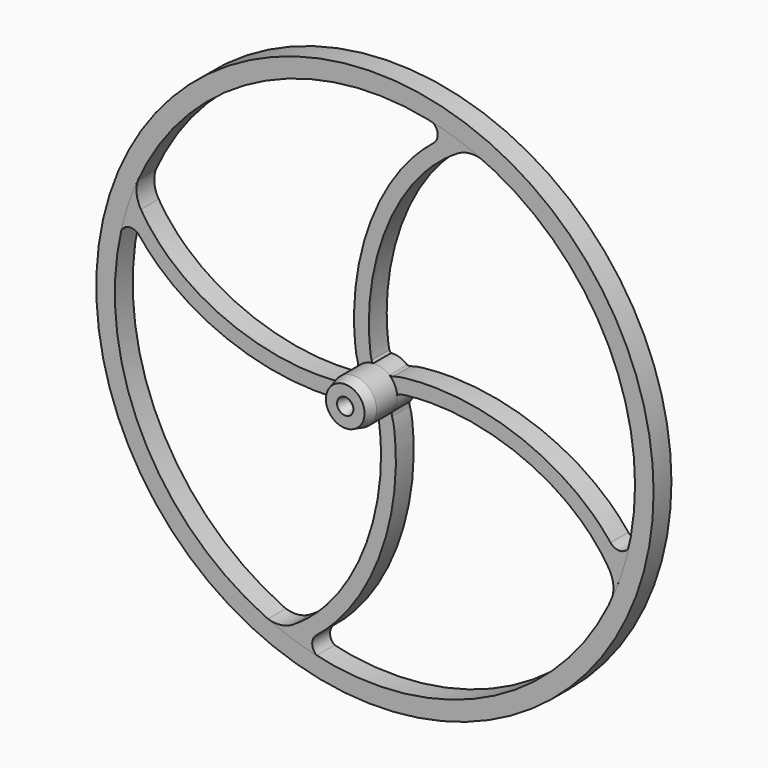
from build123d import *

# Parameters (mm, degrees)
F0_R       = 37.5
F0_R_2     = 35
F1_DEPTH   = 3
F0_R_3     = 3
F0_R_4     = 0.7
F4_DEPTH   = 3
F5_COUNT   = 4
F7_R       = 3
F7_R_2     = 0.7
F8_DEPTH   = 5
F9_SIZE2   = 0.4
F9_SIZE    = 1.5
F9_2_SIZE2 = 0.4
F9_2_SIZE  = 1.5


# Not quite as in the source:
# - ends of sketch curves that miss each other by under 0.0002 mm in the source are joined
# - the dataset's text gives a spline's control points without its knots; the knots are read off the source's solid


with BuildPart() as f1:
    # F0 (on Front) → F1 (new body)
    with BuildSketch(Plane.XZ):
        Circle(F0_R)
        Circle(F0_R_2, mode=Mode.SUBTRACT)
    extrude(amount=F1_DEPTH)


with BuildPart() as f1b:
    # F0 (on Front) → F1, piece 2 (new body)
    with BuildSketch(Plane.XZ):
        Circle(F0_R_3)
        Circle(F0_R_4, mode=Mode.SUBTRACT)
    extrude(amount=F1_DEPTH)


with BuildPart() as f4:
    # F3 (on face) → F4 (new body)
    with BuildSketch(Plane.XZ.offset(3)):
        with BuildLine():
            ThreePointArc((-2.4280868551, 1.6309565365), (-2.2872153637, 1.8232583141), (-2.1311526452, 2.0034503745))
            add(Edge.make_bspline(
                [(-2.1311526452, 2.0034503745), (-2.1977065405, 2.1717444924), (-2.2549931482, 2.3326503551), (-2.3048423501, 2.4901803988)],
                knots=[0, 0, 0, 0, 0.0288902622, 0.0288902622, 0.0288902622, 0.0288902622], degree=3))
            ThreePointArc((-2.3048423501, 2.4901803988), (-2.2683770897, 2.0464990877), (-2.4280868551, 1.6309565365))
        make_face()
        with BuildLine():
            add(Edge.make_bspline(
                [(-2.1311526452, 2.0034503745), (-2.1977065405, 2.1717444924), (-2.2549931482, 2.3326503551), (-2.3048423501, 2.4901803988)],
                knots=[0, 0, 0, 0, 0.0288902622, 0.0288902622, 0.0288902622, 0.0288902622], degree=3))
            ThreePointArc((-2.1311526452, 2.0034503745), (-1.1507363528, 2.6891319875), (0.0222007297, 2.9249157471))
            ThreePointArc((0.0222007297, 2.9249157471), (-0.2800742324, 3.029556036), (-0.4570654864, 3.2960027264))
            add(Edge.make_bspline(
                [(-0.4570654864, 3.2960027264), (-0.4727178572, 3.3545137562), (-0.515680271, 3.5297500391), (-0.5749840783, 3.8428284047), (-0.6360659448, 4.3062576915), (-0.6958595922, 4.889567905), (-0.7486087876, 5.5408021586), (-0.7898000894, 6.2624574416), (-0.8233073378, 7.3079898539), (-0.8141880534, 8.7588610419), (-0.6853474192, 10.6819332677), (-0.4096669774, 12.7634491557), (0.1778491607, 15.6956463237), (1.1333171686, 18.7851299849), (2.530999399, 21.8884585446), (4.2371866919, 24.9336280212), (6.8816709176, 28.3784867902), (9.5916152726, 30.5968228929), (11.0496913428, 31.4965632769)],
                knots=[0.046812209, 0.046812209, 0.046812209, 0.046812209, 0.0625, 0.09375, 0.125, 0.15625, 0.1875, 0.21875, 0.25, 0.3125, 0.375, 0.4375, 0.5, 0.625, 0.6875, 0.75, 0.875, 0.9909875528, 0.9909875528, 0.9909875528, 0.9909875528], degree=3))
            ThreePointArc((11.0496913428, 31.4965632769), (12.7185960162, 32.0691948071), (14.4715085769, 31.8680943815))
            ThreePointArc((14.4715085769, 31.8680943815), (12.4486505743, 32.7113298244), (10.3769836941, 33.4263101376))
            add(Edge.make_bspline(
                [(7.8736479572, 31.7059260755), (8.65746067, 32.3276666611), (9.4912706856, 32.9043722207), (10.3769836941, 33.4263101376)],
                knots=[0.9371130744, 0.9371130744, 0.9371130744, 0.9371130744, 1, 1, 1, 1], degree=3))
            add(Edge.make_bspline(
                [(-2.3048423501, 2.4901803988), (-2.4890381702, 3.0722634504), (-2.7337246035, 4.6590846092), (-3.053162866, 10.425761995), (-0.9601088151, 20.9968340608), (4.2354046977, 28.8199771014), (7.8736479572, 31.7059260755)],
                knots=[0.0288902622, 0.0288902622, 0.0288902622, 0.0288902622, 0.1356415306, 0.3449311024, 0.6452092441, 0.9371130744, 0.9371130744, 0.9371130744, 0.9371130744], degree=3))
        make_face()
        with BuildLine():
            ThreePointArc((7.7810678528, 34.124111462), (8.4403694224, 32.9384878835), (7.8736479572, 31.7059260755))
            add(Edge.make_bspline(
                [(7.8736479572, 31.7059260755), (8.65746067, 32.3276666611), (9.4912706856, 32.9043722207), (10.3769836941, 33.4263101376)],
                knots=[0.9371130744, 0.9371130744, 0.9371130744, 0.9371130744, 1, 1, 1, 1], degree=3))
            ThreePointArc((10.3769836941, 33.4263101376), (9.0857273054, 33.80014141), (7.7810678528, 34.124111462))
        make_face()
    extrude(amount=-F4_DEPTH)


with BuildPart() as f4b:
    # F3 (on face) → F4, piece 2 (new body)
    with BuildSketch(Plane.XZ.offset(3)):
        with BuildLine():
            ThreePointArc((15.2035467189, 31.5254209673), (14.8462052747, 31.7152953069), (14.4715085769, 31.8680943815))
            ThreePointArc((14.4715085769, 31.8680943815), (14.8385168723, 31.698870911), (15.2035467189, 31.5254209673))
        make_face()
    extrude(amount=-F4_DEPTH)


with BuildPart() as f5_1:
    # F5: instance of F4
    add(f4.part.rotate(Axis((0, -3, 0), (0, -1, 0)), 1 * 360 / F5_COUNT))


with BuildPart() as f5_2:
    # F5: instance of F4
    add(f4.part.rotate(Axis((0, -3, 0), (0, -1, 0)), 2 * 360 / F5_COUNT))


with BuildPart() as f5_3:
    # F5: instance of F4
    add(f4.part.rotate(Axis((0, -3, 0), (0, -1, 0)), 3 * 360 / F5_COUNT))


with BuildPart() as f8:
    # F7 (on face) → F8 (new body)
    with BuildSketch(Plane.XZ.offset(3)):
        Circle(F7_R)
        Circle(F7_R_2, mode=Mode.SUBTRACT)
    extrude(amount=F8_DEPTH)

    # F9
    f9_edges = [f8.edges().sort_by_distance(p)[0] for p in [
        (-0.7, -8, 0),
    ]]
    f9_side = f8.faces().sort_by_distance((-0.7, -5.5, 0))[0]
    chamfer(f9_edges, length=F9_SIZE, length2=F9_SIZE2, reference=f9_side)

    # F9#2
    f9_2_edges = [f8.edges().sort_by_distance(p)[0] for p in [
        (-3, -8, 0),
    ]]
    f9_2_side = f8.faces().sort_by_distance((-3, -5.5, 0))[0]
    chamfer(f9_2_edges, length=F9_2_SIZE, length2=F9_2_SIZE2, reference=f9_2_side)


solid = Compound([f1.part, f1b.part, f4.part, f4b.part, f5_1.part, f5_2.part, f5_3.part, f8.part])
